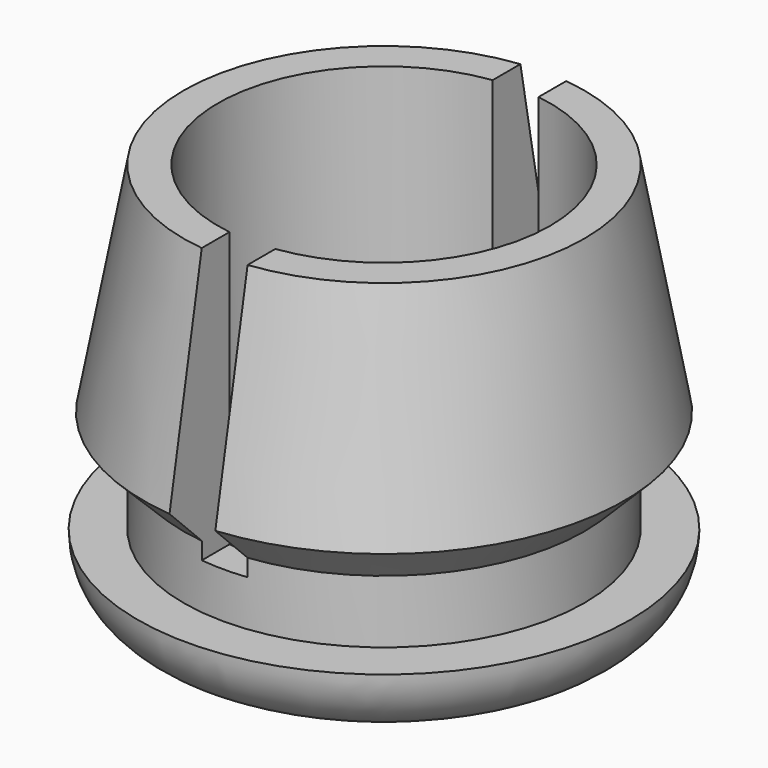
from build123d import *

# Parameters (mm, degrees)
F3_DEPTH = 12
F4_R     = 2.99999
F5_SIZE  = 1.74999


# Not quite as in the source:
# - a fillet or chamfer is up to 0.001 mm smaller than in the source, because OpenCascade refuses the exact size


with BuildPart() as f1:
    # F0 (on Front) → F1 (revolve)
    with BuildSketch(Plane.XZ):
        Polygon((0, 3), (0, 0), (10.75, 0), (10.75, 3), (8.75, 3), (8.75, 7.5), (10.5, 7.5), (8.75, 17), (7.25, 17), (7.25, 3), align=None)
    revolve(axis=Axis((0, 0, 1.5), (0, 0, 1)))

    # F2 (on face) → F3 (cut, through all)
    with BuildSketch(Plane.XY.offset(17)):
        with BuildLine():
            Line((1, -7.1807033082), (1, 7.1807033082))
            ThreePointArc((1, 7.1807033082), (0, 7.25), (-1, 7.1807033082))
            Line((-1, 7.1807033082), (-1, -7.1807033082))
            ThreePointArc((-1, -7.1807033082), (0, -7.25), (1, -7.1807033082))
        make_face()
        with BuildLine():
            Line((1, 7.1807033082), (1, 8.6926693254))
            ThreePointArc((1, 8.6926693254), (0, 8.75), (-1, 8.6926693254))
            Line((-1, 8.6926693254), (-1, 7.1807033082))
            ThreePointArc((-1, 7.1807033082), (0, 7.25), (1, 7.1807033082))
        make_face()
        with BuildLine():
            Line((-1, -7.1807033082), (-1, -8.6926693254))
            ThreePointArc((-1, -8.6926693254), (0, -8.75), (1, -8.6926693254))
            Line((1, -8.6926693254), (1, -7.1807033082))
            ThreePointArc((1, -7.1807033082), (0, -7.25), (-1, -7.1807033082))
        make_face()
        with BuildLine():
            ThreePointArc((1, -8.6926693254), (0, -8.75), (-1, -8.6926693254))
            Line((-1, -8.6926693254), (-1, -25))
            Line((-1, -25), (1, -25))
            Line((1, -25), (1, -8.6926693254))
        make_face()
        with BuildLine():
            Line((1, 8.6926693254), (1, 25))
            Line((1, 25), (-1, 25))
            Line((-1, 25), (-1, 8.6926693254))
            ThreePointArc((-1, 8.6926693254), (0, 8.75), (1, 8.6926693254))
        make_face()
    extrude(amount=-F3_DEPTH, mode=Mode.SUBTRACT)

    # F4 (radius 3 in the source; OpenCascade refuses exactly that, so slightly less here)
    f4_edges = [f1.edges().sort_by_distance(p)[0] for p in [
        (-10.75, 0, 0),
    ]]
    fillet(f4_edges, radius=F4_R)

    # F5 (size 1.75 in the source; OpenCascade refuses exactly that, so slightly less here)
    f5_edges = [f1.edges().sort_by_distance(p)[0] for p in [
        (-8.75, 0, 7.5),
        (6.531175, 5.822907, 7.5),
        (6.531175, -5.822907, 7.5),
    ]]
    chamfer(f5_edges, length=F5_SIZE)


solid = f1.part
